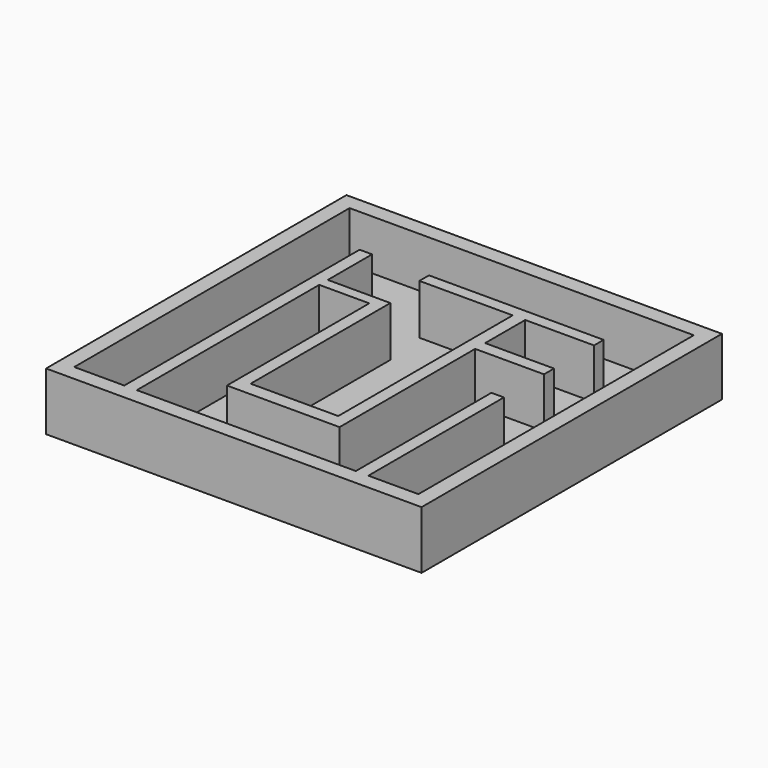
from build123d import *

# Parameters (mm, degrees)
F0_W      = 38.1
F0_H      = 38.1
F1_DEPTH  = 0.79375
F2_W      = 38.1
F2_H      = 38.1
F2_W_2    = 34.925
F2_H_2    = 34.925
F3_DEPTH  = 5.08
F4_W      = 1.27
F4_H      = 29.845
F5_DEPTH  = 5.08
F6_R      = 1.27
F7_DEPTH  = 0.396875
F9_DEPTH  = 5.08
F8_W      = 1.27
F8_H      = 17.1959060269
F10_DEPTH = 5.08
F8_R      = 1.27
F11_DEPTH = 0.396875
F8_W_2    = 6.985
F8_H_2    = 1.27
F12_DEPTH = 5.08


# Not quite as in the source:
# - a feature names something its author has since deleted; it is built from what else it names


with BuildPart() as f1:
    # F0 (on Top) → F1 (new body)
    with BuildSketch(Plane.XY):
        with Locations((-16.4964904517, -15.5271535208)):
            Rectangle(F0_W, F0_H)
    extrude(amount=F1_DEPTH)

    # F2 (on face) → F3 (join)
    with BuildSketch(Plane.XY.offset(0.79375)):
        with Locations((-16.4964904517, -15.5271535208)):
            Rectangle(F2_W, F2_H)
        with Locations((-16.4964904517, -15.5271535208)):
            Rectangle(F2_W_2, F2_H_2, mode=Mode.SUBTRACT)
    extrude(amount=F3_DEPTH)

    # F4 (on face) → F5 (join)
    with BuildSketch(Plane.XY.offset(0.79375)):
        with Locations((-28.2439904517, -18.0671535208)):
            Rectangle(F4_W, F4_H)
    extrude(amount=F5_DEPTH)

    # F6 (on face) → F7 (cut)
    with BuildSketch(Plane.XY.offset(0.79375)):
        with Locations((-31.4189904517, -30.6663066149)):
            Circle(F6_R)
    extrude(amount=-F7_DEPTH, mode=Mode.SUBTRACT)

    # F8 (on face) → F9 (join)
    with BuildSketch(Plane.XY.offset(0.79375)):
        Polygon((-4.1139904517, -3.1446535208), (-21.8377289305, -3.1446535208), (-21.8377289305, -4.3637474939), (-12.3689904517, -4.3637474939), (-12.3689904517, -26.4913998544), (-21.2589904517, -26.4913998544), (-21.2589904517, -8.7657477707), (-22.5289904517, -8.7657477707), (-27.6089904517, -8.7657477707), (-27.6089904517, -9.8523776978), (-22.5289904517, -9.8523776978), (-22.5289904517, -27.9096535208), (-11.0989904517, -27.9096535208), (-11.0989904517, -10.7137474939), (-11.0989904517, -9.4437474939), (-11.0989904517, -4.3637474939), (-4.1139904517, -4.3637474939), align=None)
    extrude(amount=F9_DEPTH)

    # F8 (on face) → F10 (join)
    with BuildSketch(Plane.XY.offset(0.79375)):
        with Locations((-4.7489904517, -24.3917005073)):
            Rectangle(F8_W, F8_H)
    extrude(amount=F10_DEPTH)

    # F8 (on face) → F11 (cut)
    with BuildSketch(Plane.XY.offset(0.79375)):
        with Locations((-25.0689904517, -13.1018003449)):
            Circle(F8_R)
    extrude(amount=-F11_DEPTH, mode=Mode.SUBTRACT)

    # F8 (on face) → F12 (join)
    with BuildSketch(Plane.XY.offset(0.79375)):
        with Locations((-7.6064904517, -10.0787474939)):
            Rectangle(F8_W_2, F8_H_2)
    extrude(amount=F12_DEPTH)


solid = f1.part
